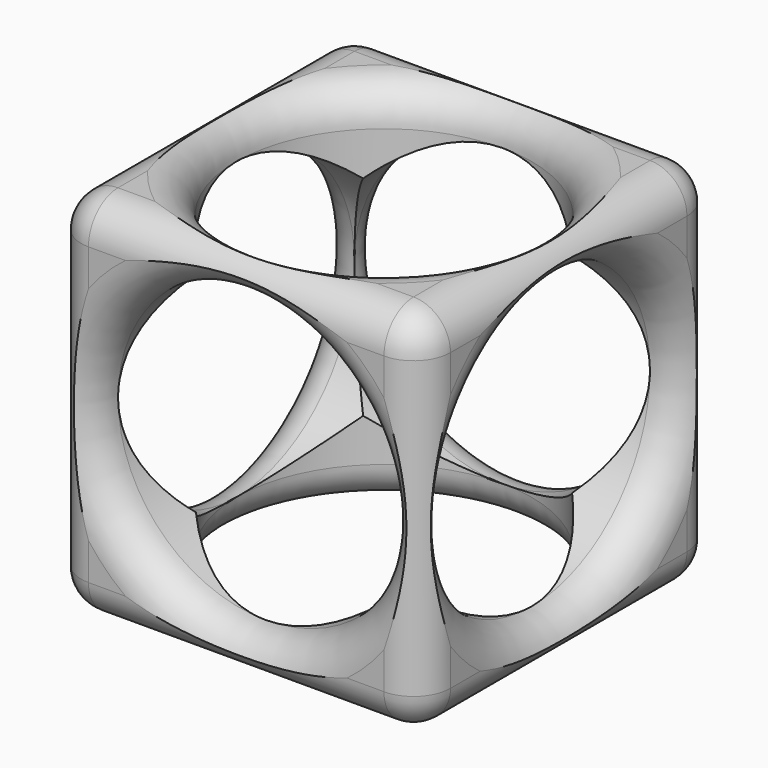
from build123d import *

# Parameters (mm, degrees)
F0_W         = 50
F0_H         = 50
F1_DEPTH     = 50
F2_R         = 20
F3_DEPTH     = 50
F4_R         = 20
F5_DEPTH     = 50
F6_R         = 20
F7_DEPTH     = 50
F8_T1_DEPTH  = 40
F8_T3_DEPTH  = 40
F8_T5_DEPTH  = 40
F8_S9_W      = 5
F8_S9_H      = 5
F8_T10_DEPTH = 5
F8_S15_W     = 5
F8_S15_H     = 5
F8_T16_DEPTH = 5
F8_S21_W     = 5
F8_S21_H     = 5
F8_T22_DEPTH = 5
F8_S27_W     = 5
F8_S27_H     = 5
F8_T28_DEPTH = 5
F8_S33_W     = 5
F8_S33_H     = 5
F8_T34_DEPTH = 5
F8_S39_W     = 5
F8_S39_H     = 5
F8_T40_DEPTH = 5
F8_S45_W     = 5
F8_S45_H     = 5
F8_T46_DEPTH = 5
F8_S51_W     = 5
F8_S51_H     = 5
F8_T52_DEPTH = 5


# Not quite as in the source:
# - a fillet or chamfer that OpenCascade refuses, or shapes differently, is made with other operations: its cross-section is extruded or revolved along the edge and cut away or added


with BuildPart() as f1:
    # F0 (on Top) → F1 (new body)
    with BuildSketch(Plane.XY):
        with Locations((25, 25)):
            Rectangle(F0_W, F0_H)
    extrude(amount=F1_DEPTH)

    # F2 (on face) → F3 (cut)
    with BuildSketch(Plane.XZ):
        with Locations((25, 25)):
            Circle(F2_R)
    extrude(amount=-F3_DEPTH, mode=Mode.SUBTRACT)

    # F4 (on face) → F5 (cut)
    with BuildSketch(Plane.YZ.offset(50)):
        with Locations((25, 25)):
            Circle(F4_R)
    extrude(amount=-F5_DEPTH, mode=Mode.SUBTRACT)

    # F6 (on face) → F7 (cut)
    with BuildSketch(Plane.XY.offset(50)):
        with Locations((25, 25)):
            Circle(F6_R)
    extrude(amount=-F7_DEPTH, mode=Mode.SUBTRACT)

    # F8: fillet of radius 5 on 18 edges, made by hand

    # F8_s2 → F8_t1 (cut)
    with BuildSketch(Plane.XZ.offset(-45)):
        with BuildLine():
            ThreePointArc((0, 45), (1.4644660941, 48.5355339059), (5, 50))
            Line((5, 50), (0, 50))
            Line((0, 50), (0, 45))
        make_face()
        with BuildLine():
            ThreePointArc((45, 50), (48.5355339059, 48.5355339059), (50, 45))
            Line((50, 45), (50, 50))
            Line((50, 50), (45, 50))
        make_face()
        with BuildLine():
            ThreePointArc((45, 0), (48.5355339059, 1.4644660941), (50, 5))
            Line((50, 5), (50, 0))
            Line((50, 0), (45, 0))
        make_face()
        with BuildLine():
            ThreePointArc((0, 5), (1.4644660941, 1.4644660941), (5, 0))
            Line((5, 0), (0, 0))
            Line((0, 0), (0, 5))
        make_face()
    extrude(amount=F8_T1_DEPTH, mode=Mode.SUBTRACT)

    # F8_s4 → F8_t3 (cut)
    with BuildSketch(Plane.YZ.offset(5)):
        with BuildLine():
            ThreePointArc((50, 45), (48.5355339059, 48.5355339059), (45, 50))
            Line((45, 50), (50, 50))
            Line((50, 50), (50, 45))
        make_face()
        with BuildLine():
            ThreePointArc((5, 50), (1.4644660941, 48.5355339059), (0, 45))
            Line((0, 45), (0, 50))
            Line((0, 50), (5, 50))
        make_face()
        with BuildLine():
            ThreePointArc((5, 0), (1.4644660941, 1.4644660941), (0, 5))
            Line((0, 5), (0, 0))
            Line((0, 0), (5, 0))
        make_face()
        with BuildLine():
            ThreePointArc((50, 5), (48.5355339059, 1.4644660941), (45, 0))
            Line((45, 0), (50, 0))
            Line((50, 0), (50, 5))
        make_face()
    extrude(amount=F8_T3_DEPTH, mode=Mode.SUBTRACT)

    # F8_s6 → F8_t5 (cut)
    with BuildSketch(Plane.XY.offset(5)):
        with BuildLine():
            ThreePointArc((45, 0), (48.5355339059, 1.4644660941), (50, 5))
            Line((50, 5), (50, 0))
            Line((50, 0), (45, 0))
        make_face()
        with BuildLine():
            ThreePointArc((45, 50), (48.5355339059, 48.5355339059), (50, 45))
            Line((50, 45), (50, 50))
            Line((50, 50), (45, 50))
        make_face()
        with BuildLine():
            ThreePointArc((0, 5), (1.4644660941, 1.4644660941), (5, 0))
            Line((5, 0), (0, 0))
            Line((0, 0), (0, 5))
        make_face()
        with BuildLine():
            ThreePointArc((0, 45), (1.4644660941, 48.5355339059), (5, 50))
            Line((5, 50), (0, 50))
            Line((0, 50), (0, 45))
        make_face()
    extrude(amount=F8_T5_DEPTH, mode=Mode.SUBTRACT)


with BuildPart() as f8_tool8:
    # F8_s9 → F8_t10 (new body)
    with BuildSketch(Plane.YZ.offset(5)):
        with Locations((47.5, 47.5)):
            Rectangle(F8_S9_W, F8_S9_H)
    extrude(amount=-F8_T10_DEPTH)

    # F8_s11 → F8_t12 (revolve, cut)
    with BuildSketch(Plane(origin=(5, 45, 45), x_dir=(0, -0.7071067812, -0.7071067812), z_dir=(0, 0.7071067812, -0.7071067812))):
        with BuildLine():
            ThreePointArc((0, -5), (5, 0), (0, 5))
            Line((0, 5), (0, -5))
        make_face()
    revolve(axis=Axis((5, 45, 45), (-1, 0, 0)), mode=Mode.SUBTRACT)


with BuildPart() as f1_1:
    add(f1.part)

    # F8_t7: cut F8_tool8
    add(f8_tool8.part, mode=Mode.SUBTRACT)


with BuildPart() as f8_tool14:
    # F8_s15 → F8_t16 (new body)
    with BuildSketch(Plane.YZ.offset(5)):
        with Locations((2.5, 47.5)):
            Rectangle(F8_S15_W, F8_S15_H)
    extrude(amount=-F8_T16_DEPTH)

    # F8_s17 → F8_t18 (revolve, cut)
    with BuildSketch(Plane(origin=(5, 5, 45), x_dir=(0, 0.7071067812, -0.7071067812), z_dir=(0, 0.7071067812, 0.7071067812))):
        with BuildLine():
            ThreePointArc((0, -5), (5, 0), (0, 5))
            Line((0, 5), (0, -5))
        make_face()
    revolve(axis=Axis((5, 5, 45), (-1, 0, 0)), mode=Mode.SUBTRACT)


with BuildPart() as f1_2:
    add(f1_1.part)

    # F8_t13: cut F8_tool14
    add(f8_tool14.part, mode=Mode.SUBTRACT)


with BuildPart() as f8_tool20:
    # F8_s21 → F8_t22 (new body)
    with BuildSketch(Plane.XZ.offset(-45)):
        with Locations((47.5, 47.5)):
            Rectangle(F8_S21_W, F8_S21_H)
    extrude(amount=-F8_T22_DEPTH)

    # F8_s23 → F8_t24 (revolve, cut)
    with BuildSketch(Plane(origin=(45, 45, 45), x_dir=(-0.7071067812, 0, -0.7071067812), z_dir=(0.7071067812, 0, -0.7071067812))):
        with BuildLine():
            ThreePointArc((0, -5), (5, 0), (0, 5))
            Line((0, 5), (0, -5))
        make_face()
    revolve(axis=Axis((45, 45, 45), (0, 1, 0)), mode=Mode.SUBTRACT)


with BuildPart() as f1_3:
    add(f1_2.part)

    # F8_t19: cut F8_tool20
    add(f8_tool20.part, mode=Mode.SUBTRACT)


with BuildPart() as f8_tool26:
    # F8_s27 → F8_t28 (new body)
    with BuildSketch(Plane.XY.offset(45)):
        with Locations((47.5, 2.5)):
            Rectangle(F8_S27_W, F8_S27_H)
    extrude(amount=F8_T28_DEPTH)

    # F8_s29 → F8_t30 (revolve, cut)
    with BuildSketch(Plane(origin=(45, 5, 45), x_dir=(-0.7071067812, 0.7071067812, 0), z_dir=(0.7071067812, 0.7071067812, 0))):
        with BuildLine():
            ThreePointArc((0, -5), (5, 0), (0, 5))
            Line((0, 5), (0, -5))
        make_face()
    revolve(axis=Axis((45, 5, 45), (0, 0, 1)), mode=Mode.SUBTRACT)


with BuildPart() as f1_4:
    add(f1_3.part)

    # F8_t25: cut F8_tool26
    add(f8_tool26.part, mode=Mode.SUBTRACT)


with BuildPart() as f8_tool32:
    # F8_s33 → F8_t34 (new body)
    with BuildSketch(Plane.XY.offset(5)):
        with Locations((47.5, 2.5)):
            Rectangle(F8_S33_W, F8_S33_H)
    extrude(amount=-F8_T34_DEPTH)

    # F8_s35 → F8_t36 (revolve, cut)
    with BuildSketch(Plane(origin=(45, 5, 5), x_dir=(-0.7071067812, 0.7071067812, 0), z_dir=(-0.7071067812, -0.7071067812, 0))):
        with BuildLine():
            ThreePointArc((0, -5), (5, 0), (0, 5))
            Line((0, 5), (0, -5))
        make_face()
    revolve(axis=Axis((45, 5, 5), (0, 0, -1)), mode=Mode.SUBTRACT)


with BuildPart() as f1_5:
    add(f1_4.part)

    # F8_t31: cut F8_tool32
    add(f8_tool32.part, mode=Mode.SUBTRACT)


with BuildPart() as f8_tool38:
    # F8_s39 → F8_t40 (new body)
    with BuildSketch(Plane.XZ.offset(-45)):
        with Locations((47.5, 2.5)):
            Rectangle(F8_S39_W, F8_S39_H)
    extrude(amount=-F8_T40_DEPTH)

    # F8_s41 → F8_t42 (revolve, cut)
    with BuildSketch(Plane(origin=(45, 45, 5), x_dir=(-0.7071067812, 0, 0.7071067812), z_dir=(-0.7071067812, 0, -0.7071067812))):
        with BuildLine():
            ThreePointArc((0, -5), (5, 0), (0, 5))
            Line((0, 5), (0, -5))
        make_face()
    revolve(axis=Axis((45, 45, 5), (0, 1, 0)), mode=Mode.SUBTRACT)


with BuildPart() as f1_6:
    add(f1_5.part)

    # F8_t37: cut F8_tool38
    add(f8_tool38.part, mode=Mode.SUBTRACT)


with BuildPart() as f8_tool44:
    # F8_s45 → F8_t46 (new body)
    with BuildSketch(Plane.YZ.offset(5)):
        with Locations((2.5, 2.5)):
            Rectangle(F8_S45_W, F8_S45_H)
    extrude(amount=-F8_T46_DEPTH)

    # F8_s47 → F8_t48 (revolve, cut)
    with BuildSketch(Plane(origin=(5, 5, 5), x_dir=(0, 0.7071067812, 0.7071067812), z_dir=(0, -0.7071067812, 0.7071067812))):
        with BuildLine():
            ThreePointArc((0, -5), (5, 0), (0, 5))
            Line((0, 5), (0, -5))
        make_face()
    revolve(axis=Axis((5, 5, 5), (-1, 0, 0)), mode=Mode.SUBTRACT)


with BuildPart() as f1_7:
    add(f1_6.part)

    # F8_t43: cut F8_tool44
    add(f8_tool44.part, mode=Mode.SUBTRACT)


with BuildPart() as f8_tool50:
    # F8_s51 → F8_t52 (new body)
    with BuildSketch(Plane.YZ.offset(5)):
        with Locations((47.5, 2.5)):
            Rectangle(F8_S51_W, F8_S51_H)
    extrude(amount=-F8_T52_DEPTH)

    # F8_s53 → F8_t54 (revolve, cut)
    with BuildSketch(Plane(origin=(5, 45, 5), x_dir=(0, -0.7071067812, 0.7071067812), z_dir=(0, -0.7071067812, -0.7071067812))):
        with BuildLine():
            ThreePointArc((0, -5), (5, 0), (0, 5))
            Line((0, 5), (0, -5))
        make_face()
    revolve(axis=Axis((5, 45, 5), (-1, 0, 0)), mode=Mode.SUBTRACT)


with BuildPart() as f1_8:
    add(f1_7.part)

    # F8_t49: cut F8_tool50
    add(f8_tool50.part, mode=Mode.SUBTRACT)

    # F8_s55 → F8_t56 (revolve, cut)
    with BuildSketch(Plane.XZ.offset(-25)):
        with BuildLine():
            ThreePointArc((50, 50), (46.4644660941, 48.5355339059), (45, 45))
            Line((45, 45), (45, 50))
            Line((45, 50), (50, 50))
        make_face()
    revolve(axis=Axis((25, 25, 50), (0, 0, 1)), mode=Mode.SUBTRACT)

    # F8_s57 → F8_t58 (revolve, cut)
    with BuildSketch(Plane.XY.offset(25)):
        with BuildLine():
            ThreePointArc((50, 50), (48.5355339059, 46.4644660941), (45, 45))
            Line((45, 45), (50, 45))
            Line((50, 45), (50, 50))
        make_face()
    revolve(axis=Axis((50, 25, 25), (1, 0, 0)), mode=Mode.SUBTRACT)

    # F8_s59 → F8_t60 (revolve, cut)
    with BuildSketch(Plane.XY.offset(25)):
        with BuildLine():
            ThreePointArc((50, 0), (46.4644660941, 1.4644660941), (45, 5))
            Line((45, 5), (45, 0))
            Line((45, 0), (50, 0))
        make_face()
    revolve(axis=Axis((25, 0, 25), (0, -1, 0)), mode=Mode.SUBTRACT)

    # F8_s61 → F8_t62 (revolve, cut)
    with BuildSketch(Plane.XY.offset(25)):
        with BuildLine():
            ThreePointArc((0, 50), (1.4644660941, 46.4644660941), (5, 45))
            Line((5, 45), (0, 45))
            Line((0, 45), (0, 50))
        make_face()
    revolve(axis=Axis((0, 25, 25), (1, 0, 0)), mode=Mode.SUBTRACT)

    # F8_s63 → F8_t64 (revolve, cut)
    with BuildSketch(Plane.XY.offset(25)):
        with BuildLine():
            ThreePointArc((50, 50), (46.4644660941, 48.5355339059), (45, 45))
            Line((45, 45), (45, 50))
            Line((45, 50), (50, 50))
        make_face()
    revolve(axis=Axis((25, 50, 25), (0, -1, 0)), mode=Mode.SUBTRACT)

    # F8_s65 → F8_t66 (revolve, cut)
    with BuildSketch(Plane.XZ.offset(-25)):
        with BuildLine():
            ThreePointArc((50, 0), (46.4644660941, 1.4644660941), (45, 5))
            Line((45, 5), (45, 0))
            Line((45, 0), (50, 0))
        make_face()
    revolve(axis=Axis((25, 25, 0), (0, 0, 1)), mode=Mode.SUBTRACT)


solid = f1_8.part
